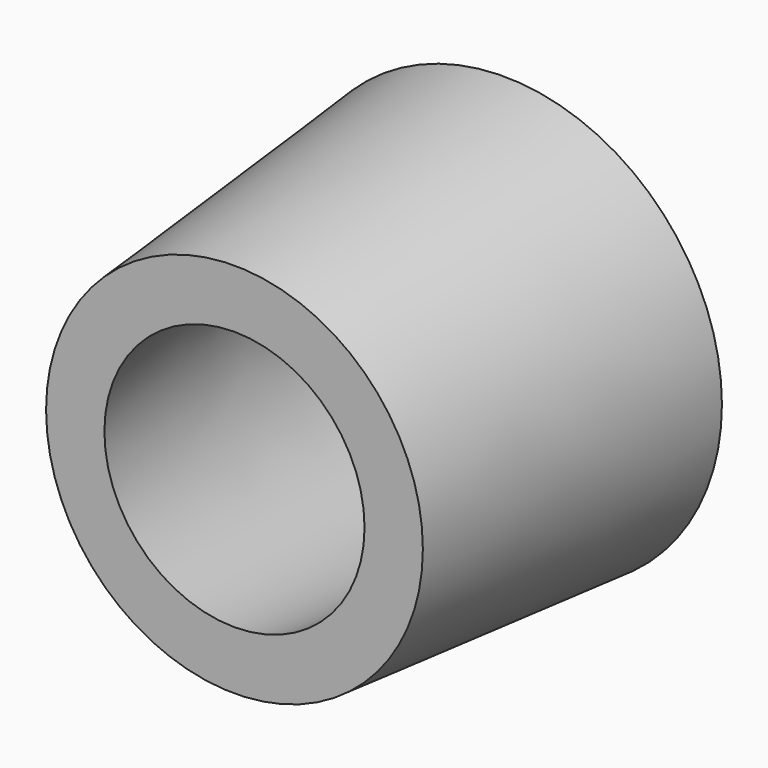
from build123d import *

# Parameters (mm, degrees)
F0_R     = 9.525
F1_DEPTH = 14.732
F1_TAPER = 5
F2_T     = -2.54


with BuildPart() as f1:
    # F0 (on Front) → F1 (new body)
    with BuildSketch(Plane.XZ):
        Circle(F0_R)
    extrude(amount=F1_DEPTH, taper=F1_TAPER)

    # F2
    f2_openings = [f1.faces().sort_by_distance(p)[0] for p in [
        (0, -14.732, 0),
        (0, 0, 0),
    ]]
    offset(amount=F2_T, openings=f2_openings, kind=Kind.INTERSECTION)


solid = f1.part
